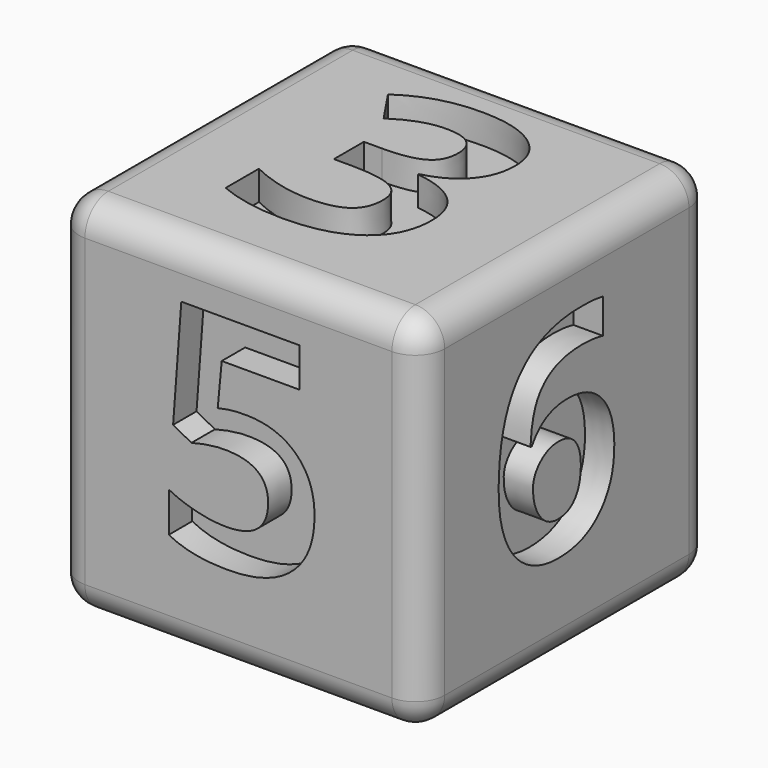
from build123d import *

# Parameters (mm, degrees)
F0_W          = 24.9381824397
F0_H          = 24.8227268457
F1_DEPTH      = 24.8
F2_TEXT_SIZE  = 21.1489923661
F3_DEPTH      = 2
F4_TEXT_SIZE  = 19.5707084559
F5_DEPTH      = 2
F6_TEXT_SIZE  = 22.0959611599
F7_DEPTH      = 2
F8_TEXT_SIZE  = 21.4646479839
F9_DEPTH      = 2
F10_TEXT_SIZE = 20.8333354547
F11_DEPTH     = 2
F12_TEXT_SIZE = 24.621214834
F13_DEPTH     = 2
F14_R         = 2


# Not quite as in the source:
# - Text() gives the source's letters only with a copy of the font that has no kerning and outlines rounded to 1/6400 em; it was checked with that copy


with BuildPart() as f1:
    # F0 (on Top) → F1 (new body)
    with BuildSketch(Plane.XY):
        with Locations((-9.0054546017, 12.4113634229)):
            Rectangle(F0_W, F0_H)
    extrude(amount=F1_DEPTH)

    # F2 (on face) → F3 (cut)
    with BuildSketch(Plane(origin=(-21.4745458215, 0, 0), x_dir=(0, -1, 0), z_dir=(-1, 0, 0))):
        with Locations((-20.0000014156, 6.0227275826)):
            Text('1', F2_TEXT_SIZE, font='Open Sans', font_style=FontStyle.BOLD, text_align=(TextAlign.LEFT, TextAlign.BOTTOM))
    extrude(amount=-F3_DEPTH, mode=Mode.SUBTRACT)

    # F4 (on face) → F5 (cut)
    with BuildSketch(Plane.YZ.offset(3.4636366181)):
        with Locations((5.9090885334, 6.4772726037)):
            Text('6', F4_TEXT_SIZE, font='Open Sans', font_style=FontStyle.BOLD, text_align=(TextAlign.LEFT, TextAlign.BOTTOM))
    extrude(amount=-F5_DEPTH, mode=Mode.SUBTRACT)

    # F6 (on face) → F7 (cut)
    with BuildSketch(Plane.XY.offset(24.8)):
        with Locations((-15.681819059, 5.5681825615)):
            Text('3', F6_TEXT_SIZE, font='Open Sans', font_style=FontStyle.BOLD, text_align=(TextAlign.LEFT, TextAlign.BOTTOM))
    extrude(amount=-F7_DEPTH, mode=Mode.SUBTRACT)

    # F8 (on face) → F9 (cut)
    with BuildSketch(Plane(origin=(0, 24.8227268457, 0), x_dir=(-1, 0, 0), z_dir=(0, 1, 0))):
        with Locations((2.7272715233, 5.5681830272)):
            Text('2', F8_TEXT_SIZE, font='Open Sans', font_style=FontStyle.BOLD, text_align=(TextAlign.LEFT, TextAlign.BOTTOM))
    extrude(amount=-F9_DEPTH, mode=Mode.SUBTRACT)

    # F10 (on face) → F11 (cut)
    with BuildSketch(Plane.XZ):
        with Locations((-14.7727280855, 6.2500005588)):
            Text('5', F10_TEXT_SIZE, font='Open Sans', font_style=FontStyle.BOLD, text_align=(TextAlign.LEFT, TextAlign.BOTTOM))
    extrude(amount=-F11_DEPTH, mode=Mode.SUBTRACT)

    # F12 (on face) → F13 (cut)
    with BuildSketch(Plane(origin=(0, 0, 0), x_dir=(1, 0, 0), z_dir=(0, 0, -1))):
        with Locations((-15.9090925008, -21.2500020862)):
            Text('4', F12_TEXT_SIZE, font='Open Sans', font_style=FontStyle.BOLD, text_align=(TextAlign.LEFT, TextAlign.BOTTOM))
    extrude(amount=-F13_DEPTH, mode=Mode.SUBTRACT)

    # F14
    f14_edges = [f1.edges().sort_by_distance(p)[0] for p in [
        (-9.005455, 0, 24.8),
        (3.463637, 12.411363, 24.8),
        (3.463637, 0, 12.4),
        (-9.005455, 0, 0),
        (-21.474546, 0, 12.4),
        (3.463637, 12.411363, 0),
        (-9.005455, 24.822727, 0),
        (-21.474546, 12.411363, 0),
        (3.463637, 24.822727, 12.4),
        (-21.474546, 12.411363, 24.8),
        (-21.474546, 24.822727, 12.4),
        (-9.005455, 24.822727, 24.8),
    ]]
    fillet(f14_edges, radius=F14_R)


solid = f1.part
